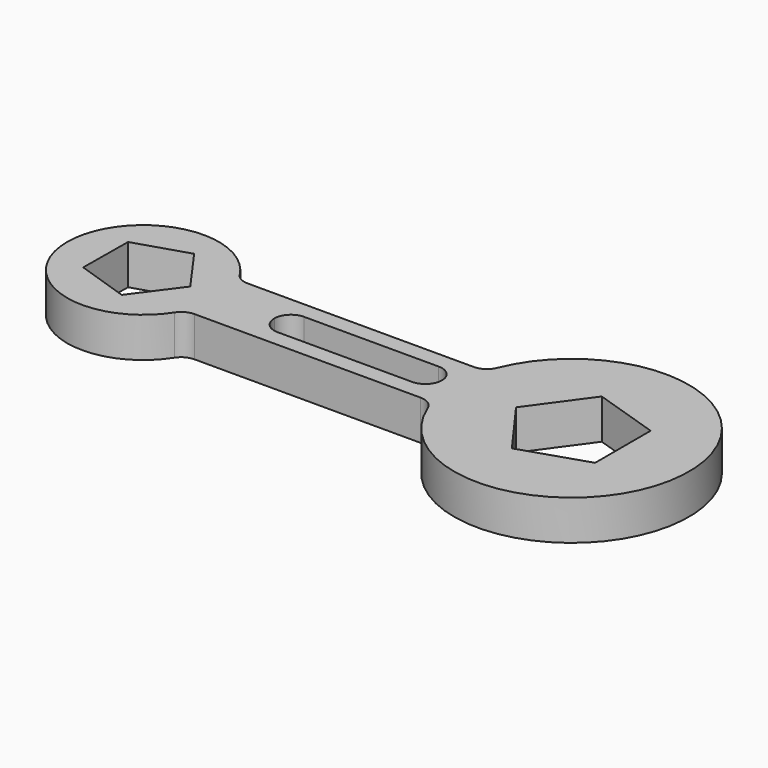
from build123d import *

# Parameters (mm, degrees)
F0_W      = 129
F0_H      = 20
F1_DEPTH  = 12
F2_R      = 22.8473442097
F4_DEPTH  = 12
F3_R      = 35.3466345688
F5_DEPTH  = 12
F6_W      = 50.4865964812
F6_H      = 10
F7_DEPTH  = 12
F8_DEPTH  = 12
F9_R      = 4.99999
F11_DEPTH = 12
F13_DEPTH = 12
F14_R     = 5


# Not quite as in the source:
# - a fillet or chamfer is up to 0.001 mm smaller than in the source, because OpenCascade refuses the exact size


with BuildPart() as f1:
    # F0 (on Top) → F1 (new body)
    with BuildSketch(Plane.XY):
        with Locations((-0.2432982406, 9.9970398602)):
            Rectangle(F0_W, F0_H)
    extrude(amount=F1_DEPTH)

    # F2 (on Top) → F4 (join)
    with BuildSketch(Plane.XY):
        with Locations((-64.7432982406, 9.9970398602)):
            Circle(F2_R)
    extrude(amount=F4_DEPTH)

    # F3 (on Top) → F5 (join)
    with BuildSketch(Plane.XY):
        with Locations((64.2567017594, 9.9970398602)):
            Circle(F3_R)
    extrude(amount=F5_DEPTH)

    # F6 (on Top) → F7 (join)
    with BuildSketch(Plane.XY):
        with Locations((0, 10)):
            Rectangle(F6_W, F6_H)
    extrude(amount=F7_DEPTH)

    # F6 (on Top) → F8 (cut)
    with BuildSketch(Plane.XY):
        with Locations((0, 10)):
            Rectangle(F6_W, F6_H)
    extrude(amount=F8_DEPTH, mode=Mode.SUBTRACT)

    # F9 (radius 5 in the source; OpenCascade refuses exactly that, so slightly less here)
    f9_edges = [f1.edges().sort_by_distance(p)[0] for p in [
        (-25.243298, 15, 6),
        (25.243298, 15, 6),
        (25.243298, 5, 6),
        (-25.243298, 5, 6),
    ]]
    fillet(f9_edges, radius=F9_R)

    # F10 (on face) → F11 (cut)
    with BuildSketch(Plane.XY):
        Polygon((-60.7340801705, -3.0663675243), (-50.8161764394, 10.3375567669), (-60.499265179, 23.9120841357), (-76.4016468673, 18.8976791396), (-76.5467705132, 2.2240790499), align=None)
    extrude(amount=F11_DEPTH, mode=Mode.SUBTRACT)

    # F12 (on face) → F13 (cut)
    with BuildSketch(Plane.XY):
        Polygon((79.5819759369, -0.3051165918), (79.5819759369, 20.6023402938), (59.6978028267, 27.0630997807), (47.4087080063, 10.148611851), (59.6978028267, -6.7658760786), align=None)
    extrude(amount=F13_DEPTH, mode=Mode.SUBTRACT)

    # F14
    f14_edges = [f1.edges().sort_by_distance(p)[0] for p in [
        (-44.200632, -0.00296, 6),
        (30.354127, -0.00296, 6),
        (30.354127, 19.99704, 6),
        (-44.200632, 19.99704, 6),
    ]]
    fillet(f14_edges, radius=F14_R)


solid = f1.part
